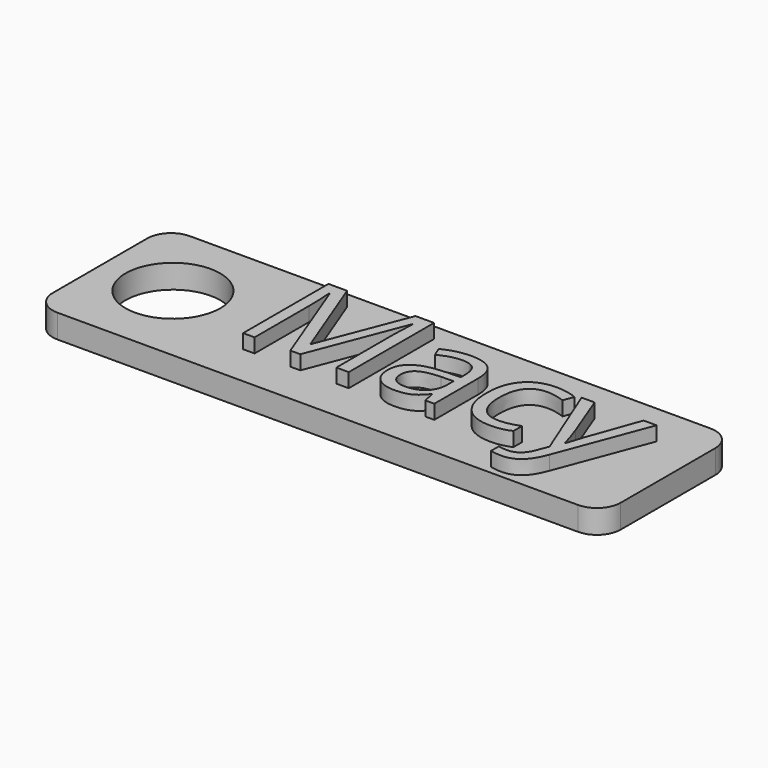
from build123d import *

# Parameters (mm, degrees)
F0_W         = 120
F0_H         = 35
F0_R         = 10
F1_DEPTH     = 5
F2_TEXT_SIZE = 31.5586687066
F3_DEPTH     = 3
F4_R         = 5


# Not quite as in the source:
# - Text() gives the source's letters only with a copy of the font that has no kerning and outlines rounded to 1/6400 em; it was checked with that copy


with BuildPart() as f1:
    # F0 (on Top) → F1 (new body)
    with BuildSketch(Plane.XY):
        with Locations((-0.8044303954, -0.5)):
            Rectangle(F0_W, F0_H)
        with Locations((-45.8044303954, 0)):
            Circle(F0_R, mode=Mode.SUBTRACT)
    extrude(amount=F1_DEPTH)

    # F2 (on face) → F3 (join)
    with BuildSketch(Plane.XY.offset(5)):
        with Locations((-26.807111688, -9.0701850131)):
            Text('Macy', F2_TEXT_SIZE, font='Open Sans', text_align=(TextAlign.LEFT, TextAlign.BOTTOM))
    extrude(amount=F3_DEPTH)

    # F4
    f4_edges = [f1.edges().sort_by_distance(p)[0] for p in [
        (59.19557, -18, 2.5),
        (59.19557, 17, 2.5),
        (-60.80443, -18, 2.5),
        (-60.80443, 17, 2.5),
    ]]
    fillet(f4_edges, radius=F4_R)


solid = f1.part
